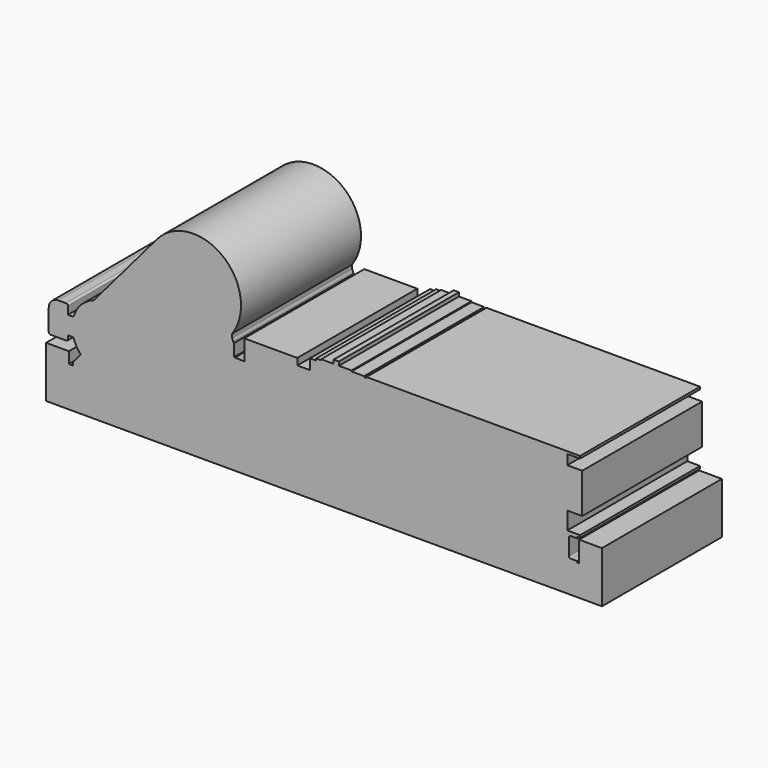
from build123d import *

# Parameters (mm, degrees)
F1_DEPTH = 1003.3


# Not quite as in the source:
# - ends of sketch curves that miss each other by under 0.0002 mm in the source are joined


with BuildPart() as f1:
    # F0 (on Front) → F1 (new body)
    with BuildSketch(Plane.XZ):
        with BuildLine():
            Line((-2939.4839356, -616.5813424), (-2939.4839356, -959.4813424))
            Line((-2939.4839356, -959.4813424), (778.4410644, -959.4813424))
            Line((778.4410644, -959.4813424), (778.4410644, -616.5813424))
            Line((778.4410644, -616.5813424), (626.0410644, -616.5813424))
            Line((626.0410644, -616.5813424), (626.0410644, -756.2813424))
            Line((626.0410644, -756.2813424), (613.264839, -756.2813424))
            Line((613.264839, -756.2813424), (613.264839, -746.7563424))
            Line((613.264839, -746.7563424), (568.8275644, -746.7563424))
            ThreePointArc((568.8275644, -746.7563424), (560.9698402941, -743.5015665059), (557.7150644, -735.6438424))
            Line((557.7150644, -735.6438424), (557.7150644, -624.5188424))
            ThreePointArc((557.7150644, -624.5188424), (560.9698402941, -616.6611182941), (568.8275644, -613.4063424))
            Line((568.8275644, -613.4063424), (613.264839, -613.4063424))
            Line((613.264839, -613.4063424), (613.264839, -603.8813424))
            Line((613.264839, -603.8813424), (632.3910644, -603.8813424))
            Line((632.3910644, -603.8813424), (632.3910644, -588.0063424))
            Line((632.3910644, -588.0063424), (546.6660644, -588.0063424))
            Line((546.6660644, -588.0063424), (546.6660644, -470.5313424))
            Line((546.6660644, -470.5313424), (646.6785644, -470.5313424))
            Line((646.6785644, -470.5313424), (646.6785644, -203.8313424))
            Line((646.6785644, -203.8313424), (546.6660644, -203.8313424))
            Line((546.6660644, -203.8313424), (546.6660644, -137.1563424))
            Line((546.6660644, -137.1563424), (632.3910644, -137.1563424))
            Line((632.3910644, -137.1563424), (632.3910644, -121.2813424))
            Line((632.3910644, -121.2813424), (-796.3589356, -121.2813424))
            Line((-796.3589356, -121.2813424), (-796.3589356, -122.8688424))
            Line((-796.3589356, -122.8688424), (-802.7089356, -129.2188424))
            Line((-802.7089356, -129.2188424), (-805.8839356, -129.2188424))
            Line((-805.8839356, -129.2188424), (-812.2339356, -122.8688424))
            Line((-812.2339356, -122.8688424), (-812.2339356, -121.2813424))
            Line((-812.2339356, -121.2813424), (-896.3714356, -121.2813424))
            Line((-896.3714356, -121.2813424), (-896.3714356, -114.9313424))
            Line((-896.3714356, -114.9313424), (-980.5089356, -114.9313424))
            Line((-980.5089356, -114.9313424), (-980.5089356, -89.5313424))
            Line((-980.5089356, -89.5313424), (-1015.4339356, -89.5313424))
            Line((-1015.4339356, -89.5313424), (-1015.4339356, -114.9313424))
            Line((-1015.4339356, -114.9313424), (-1099.5714356, -114.9313424))
            Line((-1099.5714356, -114.9313424), (-1099.5714356, -121.2813424))
            Line((-1099.5714356, -121.2813424), (-1132.9089356, -121.2813424))
            Line((-1132.9089356, -121.2813424), (-1132.9089356, -133.9813424))
            Line((-1132.9089356, -133.9813424), (-1148.7839356, -133.9813424))
            Line((-1148.7839356, -133.9813424), (-1174.1839356, -133.9813424))
            Line((-1174.1839356, -133.9813424), (-1174.1839356, -203.8313424))
            Line((-1174.1839356, -203.8313424), (-1259.05895, -203.8313424))
            Line((-1259.05895, -203.8313424), (-1259.05895, -159.3813424))
            Line((-1259.05895, -159.3813424), (-1613.699211, -159.3813424))
            Line((-1613.699211, -159.3813424), (-1613.699211, -294.3812756))
            Line((-1613.699211, -294.3812756), (-1646.1628748, -294.3812756))
            ThreePointArc((-1646.1628748, -294.3812756), (-1651.7627631889, -294.0190472383), (-1657.275348851, -292.9695922491))
            Line((-1657.275348851, -292.9695922491), (-1675.7391174, -292.9695944))
            Line((-1675.7391174, -292.9695944), (-1677.1249922, -292.169469))
            Line((-1677.1249922, -292.169469), (-1682.8014604, -292.169469))
            Line((-1682.8014604, -292.169469), (-1682.8014604, -210.4132444))
            Line((-1682.8014604, -210.4132444), (-1685.1643462, -210.4132444))
            Line((-1685.1643462, -210.4132444), (-1688.2464838, -201.946002))
            Line((-1688.2464838, -201.946002), (-1694.410124, -185.0132444))
            Line((-1694.410124, -185.0132444), (-1694.8839341458, -158.2775865747))
            ThreePointArc((-1694.8839341458, -158.2775865747), (-1758.355211766, 279.0397129741), (-2197.9610443697, 234.0759997359))
            Line((-2197.9610443697, 234.0759997359), (-2619.8151165819, -262.1438110898))
            ThreePointArc((-2619.8151165819, -262.1438110898), (-2705.0357961417, -316.4357706996), (-2755.9076582696, -403.7411814515))
            Line((-2755.9076582696, -403.7411814515), (-2793.5718559027, -404.7273278365))
            Line((-2793.5718559027, -404.7273278365), (-2793.5718559027, -353.1400729063))
            ThreePointArc((-2793.5718559027, -353.1400729063), (-2797.7147534728, -343.7557355538), (-2807.4405116, -340.493985))
            Line((-2807.4405116, -340.493985), (-2858.2403846, -340.493985))
            ThreePointArc((-2858.2403846, -340.493985), (-2903.1415574423, -359.0926597577), (-2921.7402322, -403.9938326))
            Line((-2921.7402322, -403.9938326), (-2921.7402322, -546.868477))
            ThreePointArc((-2921.7402322, -546.868477), (-2917.5973338103, -556.2528150998), (-2907.8715742938, -559.5145647022))
            Line((-2907.8715742938, -559.5145647022), (-2802.3094282938, -559.5145647022))
            ThreePointArc((-2802.3094282938, -559.5145647022), (-2796.1310300431, -556.9553883529), (-2793.5718536938, -550.7769901022))
            Line((-2793.5718536938, -550.7769901022), (-2793.5718536938, -524.4830607299))
            Line((-2793.5718536938, -524.4830607299), (-2755.9704253207, -525.4675636528))
            ThreePointArc((-2755.9704253207, -525.4675636528), (-2736.7875568064, -570.3667556741), (-2707.9399906828, -609.7588591639))
            Line((-2707.9399906828, -609.7588591639), (-2760.1328298938, -671.9575077155))
            Line((-2760.1328298938, -671.9575077155), (-2760.1328298938, -692.1022345022))
            Line((-2760.1328298938, -692.1022345022), (-2787.1466950938, -692.1022345022))
            Line((-2787.1466950938, -692.1022345022), (-2787.1466950938, -616.5813424))
            Line((-2787.1466950938, -616.5813424), (-2939.4839356, -616.5813424))
        make_face()
    extrude(amount=F1_DEPTH)


solid = f1.part
